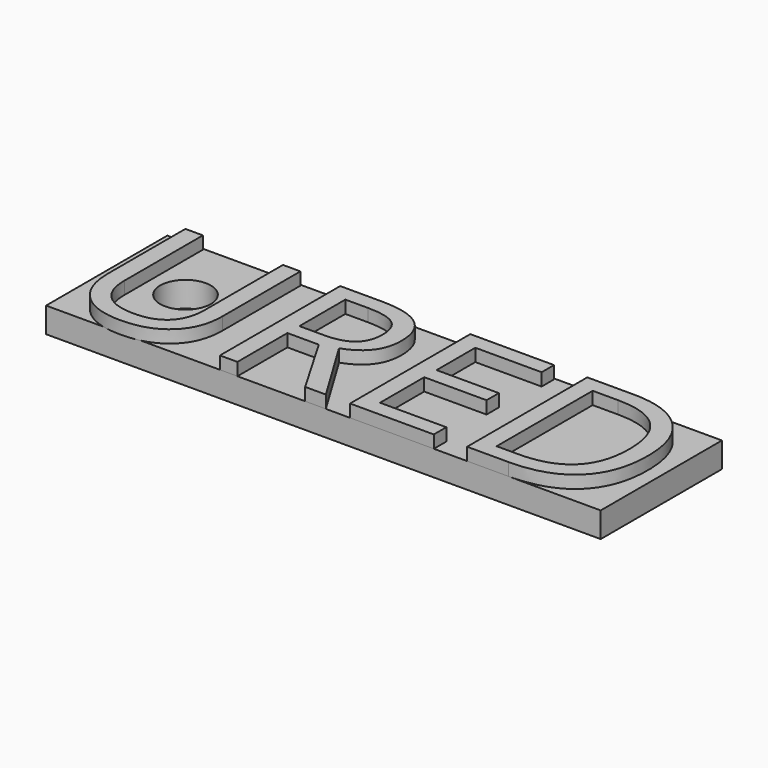
from build123d import *

# Parameters (mm, degrees)
F0_TEXT_SIZE = 16.6666666667
F2_DEPTH     = 1
F1_W         = 43.9166666667
F1_H         = 12
F3_DEPTH     = 2
F4_R         = 2
F5_DEPTH     = 2.001


# Not quite as in the source:
# - Text() gives the source's letters only with a copy of the font that has no kerning and outlines rounded to 1/6400 em; it was checked with that copy


with BuildPart() as f2:
    # F0 (on Top) → F2 (new body)
    with BuildSketch(Plane.XY):
        with Locations((-34.6995065734, 0)):
            Text('URED', F0_TEXT_SIZE, font='Open Sans', text_align=(TextAlign.LEFT, TextAlign.BOTTOM))
    extrude(amount=F2_DEPTH)


with BuildPart() as f3:
    # F1 (on Top) → F3 (new body)
    with BuildSketch(Plane.XY):
        with Locations((-12.7411732401, 6)):
            Rectangle(F1_W, F1_H)
    extrude(amount=-F3_DEPTH)

    # F4 (on face) → F5 (cut, through all)
    with BuildSketch(Plane.XY):
        with Locations((-28.8718268275, 6.5141133964)):
            Circle(F4_R)
    extrude(amount=-F5_DEPTH, mode=Mode.SUBTRACT)


solid = Compound([f2.part, f3.part])
